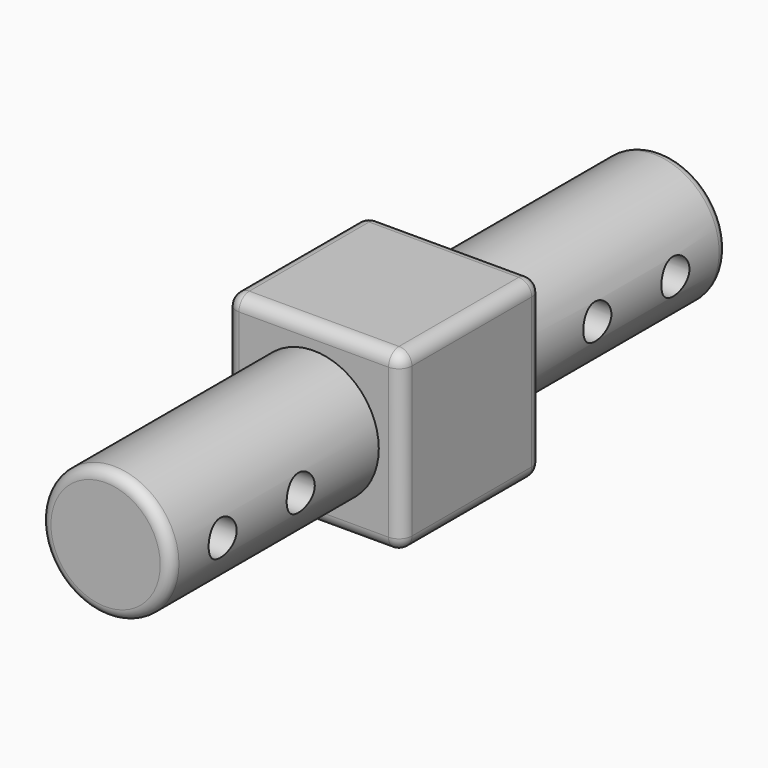
from build123d import *

# Parameters (mm, degrees)
F0_W      = 34.29
F0_H      = 34.29
F1_DEPTH  = 34.29
F3_R      = 12.7
F4_DEPTH  = 50.8
F5_R      = 3.429
F6_DEPTH  = 25.4
F7_R      = 3.429
F8_DEPTH  = 25.4
F9_R      = 3.429
F10_DEPTH = 25.4
F11_R     = 2.54
F12_R     = 12.7
F13_DEPTH = 50.8
F14_R     = 3.429
F15_DEPTH = 25.4
F16_R     = 2.032
F17_R     = 3.429
F18_DEPTH = 25.4


with BuildPart() as f1:
    # F0 (on Top) → F1 (new body)
    with BuildSketch(Plane.XY):
        with Locations((3.6728888822, 6.5610635031)):
            Rectangle(F0_W, F0_H)
    extrude(amount=F1_DEPTH)

    # F3 (on face) → F4 (join)
    with BuildSketch(Plane.XZ.offset(10.5839364969)):
        with Locations((3.6728888822, 17.145)):
            Circle(F3_R)
    extrude(amount=F4_DEPTH)

    # F5 (on Front) → F6 (cut, symmetric)
    with BuildSketch(Plane.XZ):
        with Locations((3.6728888822, 53.34)):
            Circle(F5_R)
        with Locations((3.6728888822, 72.39)):
            Circle(F5_R)
    extrude(amount=F6_DEPTH, both=True, mode=Mode.SUBTRACT)

    # F7 (on Right) → F8 (cut, symmetric)
    with BuildSketch(Plane.YZ):
        with Locations((-29.6339364969, 17.145)):
            Circle(F7_R)
        with Locations((-48.6839364969, 17.145)):
            Circle(F7_R)
    extrude(amount=F8_DEPTH, both=True, mode=Mode.SUBTRACT)

    # F9 (on Front) → F10 (cut, symmetric)
    with BuildSketch(Plane.XZ):
        with Locations((-51.5721111178, 17.145)):
            Circle(F9_R)
        with Locations((-32.5221111178, 17.145)):
            Circle(F9_R)
    extrude(amount=F10_DEPTH, both=True, mode=Mode.SUBTRACT)

    # F11
    f11_edges = [f1.edges().sort_by_distance(p)[0] for p in [
        (20.817889, 23.706064, 17.145),
        (20.817889, 6.561064, 34.29),
        (20.817889, -10.583936, 17.145),
        (20.817889, 6.561064, 0),
        (3.672889, 23.706064, 0),
        (3.672889, 23.706064, 34.29),
        (-13.472111, 23.706064, 17.145),
        (-13.472111, 6.561064, 0),
        (3.672889, -10.583936, 0),
        (-13.472111, 6.561064, 34.29),
        (-13.472111, -10.583936, 17.145),
        (3.672889, -10.583936, 34.29),
    ]]
    fillet(f11_edges, radius=F11_R)

    # F12 (on face) → F13 (join)
    with BuildSketch(Plane(origin=(0, 23.7060635031, 0), x_dir=(-1, 0, 0), z_dir=(0, 1, 0))):
        with Locations((-3.6728888822, 17.145)):
            Circle(F12_R)
    extrude(amount=F13_DEPTH)

    # F14 (on Right) → F15 (cut, symmetric)
    with BuildSketch(Plane.YZ):
        with Locations((42.7560635031, 17.145)):
            Circle(F14_R)
        with Locations((61.8060635031, 17.145)):
            Circle(F14_R)
    extrude(amount=F15_DEPTH, both=True, mode=Mode.SUBTRACT)

    # F16
    f16_edges = [f1.edges().sort_by_distance(p)[0] for p in [
        (-9.027111, -61.383936, 17.145),
        (16.372889, 74.506064, 17.145),
    ]]
    fillet(f16_edges, radius=F16_R)

    # F17 (on Front) → F18 (cut, symmetric)
    with BuildSketch(Plane.XZ):
        with Locations((58.9178888822, 17.145)):
            Circle(F17_R)
        with Locations((39.8678888822, 17.145)):
            Circle(F17_R)
    extrude(amount=F18_DEPTH, both=True, mode=Mode.SUBTRACT)


solid = f1.part
